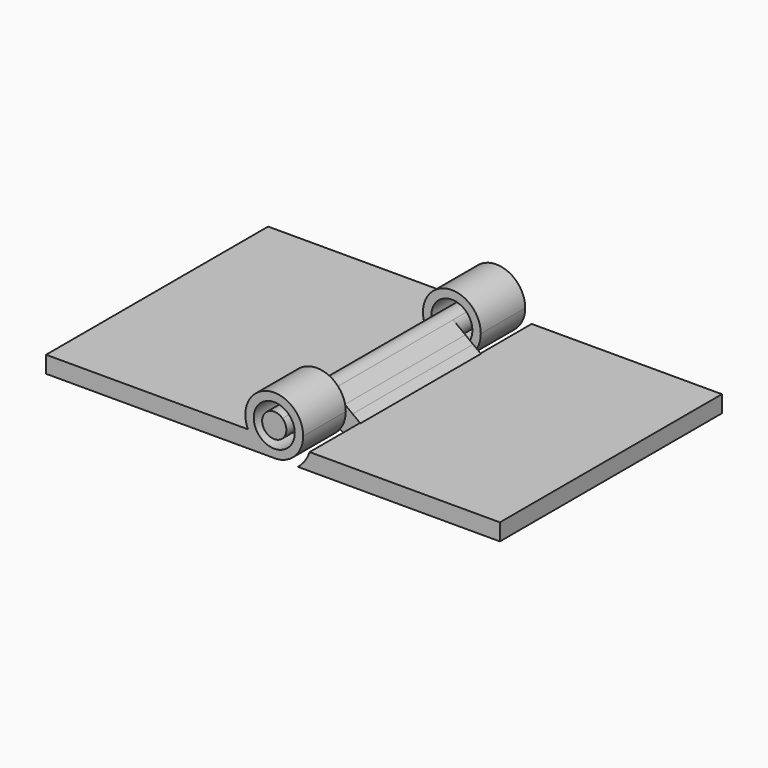
from build123d import *

# Parameters (mm, degrees)
F0_W     = 24
F0_H     = 2
F1_DEPTH = 33
F0_R     = 2.4385073591
F2_DEPTH = 6.604
F3_START = 26.67
F3_DEPTH = 6.33
F5_DEPTH = 33
F7_DEPTH = 33
F8_START = -7.6454
F8_DEPTH = 17.907


with BuildPart() as f1:
    # F0 (on Front) → F1 (new body)
    with BuildSketch(Plane.XZ):
        with Locations((-13.9121894147, 15.6936606616)):
            Rectangle(F0_W, F0_H)
        with BuildLine():
            ThreePointArc((0.9247052946, 14.6936606616), (-0.764623467, 15.3094296465), (-1.9121894147, 16.6936606616))
            Line((-1.9121894147, 16.6936606616), (-1.9121894147, 14.6936606616))
            Line((-1.9121894147, 14.6936606616), (0.9247052946, 14.6936606616))
        make_face()
    extrude(amount=F1_DEPTH)

    # F0 (on Front) → F2 (join)
    with BuildSketch(Plane.XZ):
        with BuildLine():
            ThreePointArc((4.6551508029, 18.1197524549), (0.4869798056, 21.4799494482), (-1.9121894147, 16.6936606616))
            ThreePointArc((-1.9121894147, 16.6936606616), (-0.764623467, 15.3094296465), (0.9247052946, 14.6936606616))
            Line((0.9247052946, 14.6936606616), (1.5085815929, 14.6936606616))
            ThreePointArc((1.5085815929, 14.6936606616), (3.7491485605, 15.7938653784), (4.6551508029, 18.1197524549))
        make_face()
        with Locations((1.2166434437, 18.1197524549)):
            Circle(F0_R, mode=Mode.SUBTRACT)
    extrude(amount=F2_DEPTH)

    # F0 (on Front) → F3 (join)
    with BuildSketch(Plane.XZ.offset(F3_START)):
        with BuildLine():
            ThreePointArc((4.6551508029, 18.1197524549), (0.4869798056, 21.4799494482), (-1.9121894147, 16.6936606616))
            ThreePointArc((-1.9121894147, 16.6936606616), (-0.764623467, 15.3094296465), (0.9247052946, 14.6936606616))
            Line((0.9247052946, 14.6936606616), (1.5085815929, 14.6936606616))
            ThreePointArc((1.5085815929, 14.6936606616), (3.7491485605, 15.7938653784), (4.6551508029, 18.1197524549))
        make_face()
        with Locations((1.2166434437, 18.1197524549)):
            Circle(F0_R, mode=Mode.SUBTRACT)
    extrude(amount=F3_DEPTH)


with BuildPart() as f5:
    # F4 (on face) → F5 (new body, through all)
    with BuildSketch(Plane(origin=(0, 0, 0), x_dir=(-1, 0, 0), z_dir=(0, 1, 0))):
        with BuildLine():
            Line((-15.8450398594, 14.6936606616), (-4.0383880461, 14.6936606616))
            ThreePointArc((-4.0383880461, 14.6936606616), (-4.8686763678, 15.5972530795), (-5.4198100802, 16.6936606616))
            Line((-5.4198100802, 16.6936606616), (-10.0691048428, 16.6936606616))
            Line((-10.0691048428, 16.6936606616), (-28.0413880461, 16.6936606616))
            Line((-28.0413880461, 16.6936606616), (-28.0413880461, 14.6936606616))
            Line((-28.0413880461, 14.6936606616), (-15.8450398594, 14.6936606616))
        make_face()
    extrude(amount=-F5_DEPTH)



with BuildPart() as f7:
    # F6 (on face) → F7 (new body, through all)
    with BuildSketch(Plane(origin=(0, 0, 0), x_dir=(-1, 0, 0), z_dir=(0, 1, 0))):
        with BuildLine():
            ThreePointArc((-0.3418582309, 16.9778005059), (0.073257403, 17.4829956504), (0.2218639154, 18.1197524549))
            ThreePointArc((0.2218639154, 18.1197524549), (-0.6399254334, 19.4375915038), (-2.1927219368, 19.1764332002))
            ThreePointArc((-2.1927219368, 19.1764332002), (-2.4051657689, 17.3093709984), (-0.5895183864, 16.8251414767))
            Line((-0.5895183864, 16.8251414767), (-0.3418582309, 16.9778005059))
        make_face()
    extrude(amount=-F7_DEPTH)


with BuildPart() as f5_1:
    add(f5.part)

    add(f7.part)  # F8 merges F7
    # F6 (on face) → F8 (join)
    with BuildSketch(Plane(origin=(0, 0, 0), x_dir=(-1, 0, 0), z_dir=(0, 1, 0)).offset(F8_START)):
        with BuildLine():
            ThreePointArc((-3.1272102801, 15.2608947769), (-4.0581637221, 16.1834943713), (-4.5762601156, 17.3874214661))
            Line((-4.5762601156, 17.3874214661), (-5.6122234091, 16.6098587215))
            Line((-5.6122234091, 16.6098587215), (-4.681289196, 14.9995945394))
            Line((-4.681289196, 14.9995945394), (-4.0474394336, 14.6936606616))
            Line((-4.0474394336, 14.6936606616), (-3.1272102801, 15.2608947769))
        make_face()
        with BuildLine():
            ThreePointArc((-0.5895183864, 16.8251414767), (-2.4051657689, 17.3093709984), (-2.1927219368, 19.1764332002))
            Line((-2.1927219368, 19.1764332002), (-3.6548108098, 18.0790334718))
            ThreePointArc((-3.6548108098, 18.0790334718), (-3.231770478, 16.7465877975), (-2.1464189491, 15.8654597387))
            Line((-2.1464189491, 15.8654597387), (-0.5895183864, 16.8251414767))
        make_face()
        with BuildLine():
            ThreePointArc((-2.1464189491, 15.8654597387), (-3.231770478, 16.7465877975), (-3.6548108098, 18.0790334718))
            Line((-3.6548108098, 18.0790334718), (-4.5762601156, 17.3874214661))
            ThreePointArc((-4.5762601156, 17.3874214661), (-4.0581637221, 16.1834943713), (-3.1272102801, 15.2608947769))
            Line((-3.1272102801, 15.2608947769), (-2.1464189491, 15.8654597387))
        make_face()
    extrude(amount=-F8_DEPTH)


solid = Compound([f1.part, f5_1.part])
